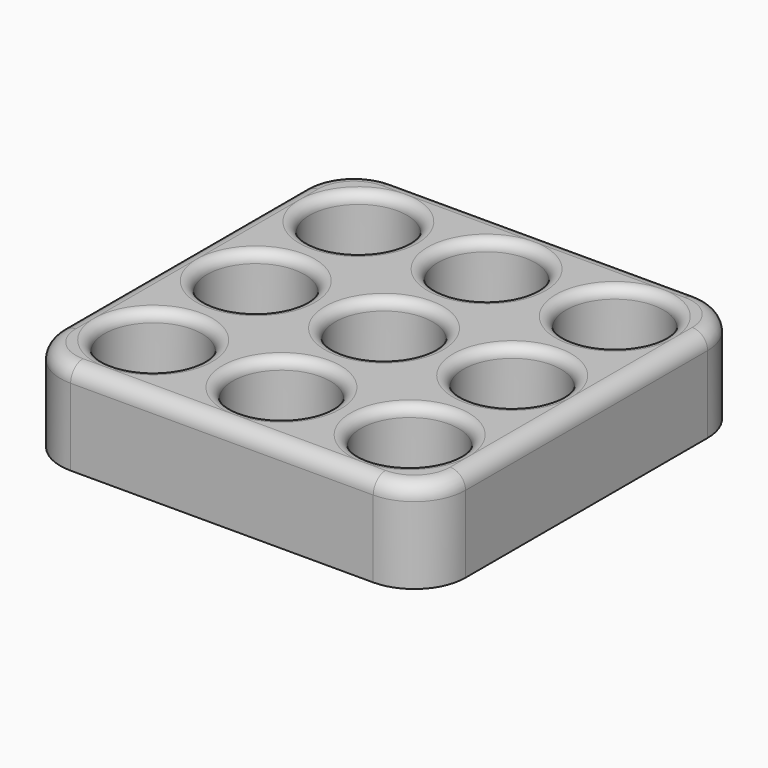
from build123d import *

# Parameters (mm, degrees)
F0_W         = 79
F0_H         = 79
F0_R         = 9.5
F1_DEPTH     = 15
F2_DEPTH     = 3
F3_R         = 3
F4_R         = 1.99999
F5_T1_DEPTH  = 43
F5_T4_ANGLE  = 90
F5_T6_ANGLE  = 90
F5_T8_ANGLE  = 90
F5_T10_ANGLE = 90


# Not quite as in the source:
# - a fillet or chamfer that OpenCascade refuses, or shapes differently, is made with other operations: its cross-section is extruded or revolved along the edge and cut away or added
# - a fillet or chamfer is up to 0.001 mm smaller than in the source, because OpenCascade refuses the exact size


with BuildPart() as f1:
    # F0 (on Top) → F1 (new body)
    with BuildSketch(Plane.XY):
        with Locations((-7.91070396, 39.5)):
            Rectangle(F0_W, F0_H)
        with Locations((-32.91070396, 14.5)):
            Circle(F0_R, mode=Mode.SUBTRACT)
        with Locations((-7.91070396, 14.5)):
            Circle(F0_R, mode=Mode.SUBTRACT)
        with Locations((17.08929604, 14.5)):
            Circle(F0_R, mode=Mode.SUBTRACT)
        with Locations((-32.91070396, 39.5)):
            Circle(F0_R, mode=Mode.SUBTRACT)
        with Locations((-32.91070396, 64.5)):
            Circle(F0_R, mode=Mode.SUBTRACT)
        with Locations((-7.91070396, 39.5)):
            Circle(F0_R, mode=Mode.SUBTRACT)
        with Locations((17.08929604, 39.5)):
            Circle(F0_R, mode=Mode.SUBTRACT)
        with Locations((-7.91070396, 64.5)):
            Circle(F0_R, mode=Mode.SUBTRACT)
        with Locations((17.08929604, 64.5)):
            Circle(F0_R, mode=Mode.SUBTRACT)
    extrude(amount=F1_DEPTH)

    # F0 (on Top) → F2 (join)
    with BuildSketch(Plane.XY):
        with Locations((-7.91070396, 39.5)):
            Rectangle(F0_W, F0_H)
        with Locations((-32.91070396, 14.5)):
            Circle(F0_R, mode=Mode.SUBTRACT)
        with Locations((-7.91070396, 14.5)):
            Circle(F0_R, mode=Mode.SUBTRACT)
        with Locations((17.08929604, 14.5)):
            Circle(F0_R, mode=Mode.SUBTRACT)
        with Locations((-32.91070396, 39.5)):
            Circle(F0_R, mode=Mode.SUBTRACT)
        with Locations((-32.91070396, 64.5)):
            Circle(F0_R, mode=Mode.SUBTRACT)
        with Locations((-7.91070396, 39.5)):
            Circle(F0_R, mode=Mode.SUBTRACT)
        with Locations((17.08929604, 39.5)):
            Circle(F0_R, mode=Mode.SUBTRACT)
        with Locations((-7.91070396, 64.5)):
            Circle(F0_R, mode=Mode.SUBTRACT)
        with Locations((17.08929604, 64.5)):
            Circle(F0_R, mode=Mode.SUBTRACT)
        with Locations((17.08929604, 64.5)):
            Circle(F0_R)
        with Locations((-7.91070396, 64.5)):
            Circle(F0_R)
        with Locations((-32.91070396, 64.5)):
            Circle(F0_R)
        with Locations((-32.91070396, 39.5)):
            Circle(F0_R)
        with Locations((-7.91070396, 39.5)):
            Circle(F0_R)
        with Locations((17.08929604, 39.5)):
            Circle(F0_R)
        with Locations((17.08929604, 14.5)):
            Circle(F0_R)
        with Locations((-7.91070396, 14.5)):
            Circle(F0_R)
        with Locations((-32.91070396, 14.5)):
            Circle(F0_R)
    extrude(amount=-F2_DEPTH)

    # F3
    f3_edges = [f1.edges().sort_by_distance(p)[0] for p in [
        (-47.410704, 39.5, 15),
        (-7.910704, 79, 15),
        (31.589296, 39.5, 15),
        (-7.910704, 0, 15),
    ]]
    fillet(f3_edges, radius=F3_R)

    # F4 (radius 2 in the source; OpenCascade refuses exactly that, so slightly less here)
    f4_edges = [f1.edges().sort_by_distance(p)[0] for p in [
        (-42.410704, 64.5, 15),
        (-17.410704, 64.5, 15),
        (7.589296, 64.5, 15),
        (7.589296, 39.5, 15),
        (7.589296, 14.5, 15),
        (-17.410704, 14.5, 15),
        (-17.410704, 39.5, 15),
        (-42.410704, 39.5, 15),
        (-42.410704, 14.5, 15),
    ]]
    fillet(f4_edges, radius=F4_R)

    # F5: fillet of radius 10 on 4 edges, made by hand

    # F5_s2 → F5_t1 (cut)
    with BuildSketch(Plane.XY.offset(-28)):
        with BuildLine():
            ThreePointArc((-47.41070396, 69), (-44.4817717719, 76.0710678119), (-37.41070396, 79))
            Line((-37.41070396, 79), (-47.41070396, 79))
            Line((-47.41070396, 79), (-47.41070396, 69))
        make_face()
        with BuildLine():
            ThreePointArc((21.58929604, 79), (28.6603638519, 76.0710678119), (31.58929604, 69))
            Line((31.58929604, 69), (31.58929604, 79))
            Line((31.58929604, 79), (21.58929604, 79))
        make_face()
        with BuildLine():
            ThreePointArc((21.58929604, 0), (28.6603638519, 2.9289321881), (31.58929604, 10))
            Line((31.58929604, 10), (31.58929604, 0))
            Line((31.58929604, 0), (21.58929604, 0))
        make_face()
        with BuildLine():
            ThreePointArc((-47.41070396, 10), (-44.4817717719, 2.9289321881), (-37.41070396, 0))
            Line((-37.41070396, 0), (-47.41070396, 0))
            Line((-47.41070396, 0), (-47.41070396, 10))
        make_face()
    extrude(amount=F5_T1_DEPTH, mode=Mode.SUBTRACT)

    # F5_s3 → F5_t4 (revolve, cut)
    with BuildSketch(Plane.XZ.offset(-10)):
        with BuildLine():
            ThreePointArc((-44.41070396, 15), (-46.5320243036, 14.1213203436), (-47.41070396, 12))
            Line((-47.41070396, 12), (-47.41070396, 15))
            Line((-47.41070396, 15), (-44.41070396, 15))
        make_face()
    revolve(axis=Axis((-37.41070396, 10, 15), (0, 0, 1)), revolution_arc=F5_T4_ANGLE, mode=Mode.SUBTRACT)

    # F5_s5 → F5_t6 (revolve, cut)
    with BuildSketch(Plane.YZ.offset(21.58929604)):
        with BuildLine():
            ThreePointArc((3, 15), (0.8786796564, 14.1213203436), (0, 12))
            Line((0, 12), (0, 15))
            Line((0, 15), (3, 15))
        make_face()
    revolve(axis=Axis((21.58929604, 10, 15), (0, 0, 1)), revolution_arc=F5_T6_ANGLE, mode=Mode.SUBTRACT)

    # F5_s7 → F5_t8 (revolve, cut)
    with BuildSketch(Plane.XZ.offset(-69)):
        with BuildLine():
            ThreePointArc((28.58929604, 15), (30.7106163836, 14.1213203436), (31.58929604, 12))
            Line((31.58929604, 12), (31.58929604, 15))
            Line((31.58929604, 15), (28.58929604, 15))
        make_face()
    revolve(axis=Axis((21.58929604, 69, 15), (0, 0, 1)), revolution_arc=F5_T8_ANGLE, mode=Mode.SUBTRACT)

    # F5_s9 → F5_t10 (revolve, cut)
    with BuildSketch(Plane.YZ.offset(-37.41070396)):
        with BuildLine():
            ThreePointArc((76, 15), (78.1213203436, 14.1213203436), (79, 12))
            Line((79, 12), (79, 15))
            Line((79, 15), (76, 15))
        make_face()
    revolve(axis=Axis((-37.41070396, 69, 15), (0, 0, 1)), revolution_arc=F5_T10_ANGLE, mode=Mode.SUBTRACT)


solid = f1.part
